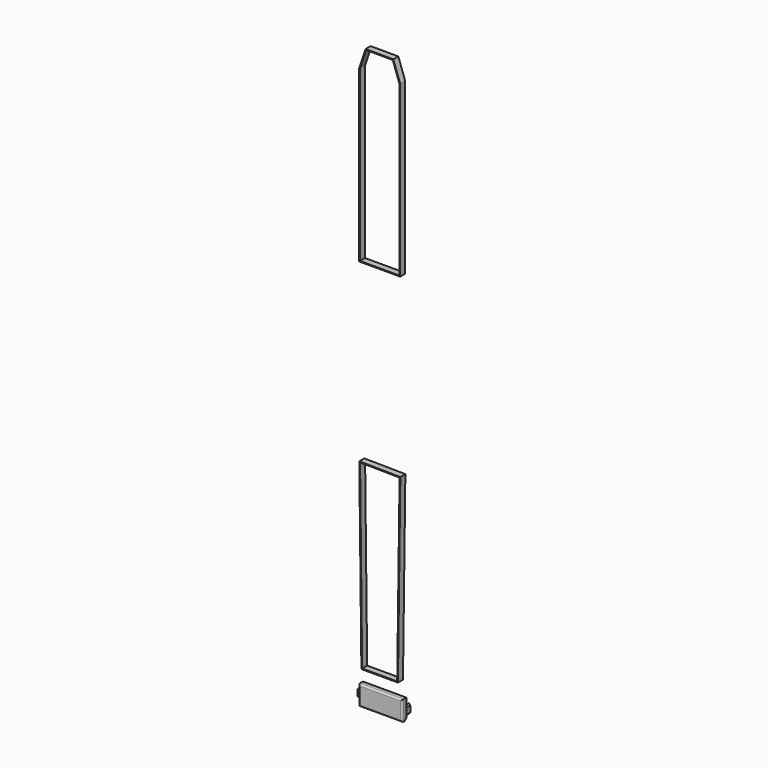
from build123d import *

# Parameters (mm, degrees)
F3_DEPTH       = 10.16
F5_DEPTH       = 10.16
F6_DEPTH       = 3.048
F7_W           = 70.5953985453
F7_H           = 32.1978032589
F8_DEPTH       = 10.16
F9_SIZE        = 5.08
F10_SIZE       = 1.778
F11_R          = 2.54
F12_T1_DEPTH   = 41.1774884869
F12_2_T1_DEPTH = 41.1774884869


# Not quite as in the source:
# - a fillet or chamfer that OpenCascade refuses, or shapes differently, is made with other operations: its cross-section is extruded or revolved along the edge and cut away or added


with BuildPart() as f3:
    # F2 (on offset) → F3 (new body)
    with BuildSketch(Plane.XZ.offset(-43.18)):
        Polygon((-35.3846980661, 135.4740036093), (30.9212480387, 135.4740036093), (30.9212480387, 410.4879885195), (19.851437657, 441.7302218888), (-0.0477681745, 441.8133852342), (-25.0969552653, 441.9180715325), (-35.3846980661, 411.4112124139), align=None)
        Polygon((29.6512480387, 410.2696444457), (29.6512480387, 136.7440036093), (-34.1146980661, 136.7440036093), (-34.1146980661, 411.2028378599), (-24.1862514864, 440.6442544017), (-0.0530757494, 440.5433963249), (18.9527356185, 440.46396668), align=None, mode=Mode.SUBTRACT)
    extrude(amount=F3_DEPTH)

    # F2 (on offset) → F6 (join)
    with BuildSketch(Plane.XZ.offset(-43.18)):
        Polygon((-35.3846980661, 135.4740036093), (30.9212480387, 135.4740036093), (30.9212480387, 410.4879885195), (19.851437657, 441.7302218888), (-0.0477681745, 441.8133852342), (-25.0969552653, 441.9180715325), (-35.3846980661, 411.4112124139), align=None)
        Polygon((29.6512480387, 410.2696444457), (29.6512480387, 136.7440036093), (-34.1146980661, 136.7440036093), (-34.1146980661, 411.2028378599), (-24.1862514864, 440.6442544017), (-0.0530757494, 440.5433963249), (18.9527356185, 440.46396668), align=None, mode=Mode.SUBTRACT)
    extrude(amount=F6_DEPTH)


with BuildPart() as f5:
    # F4 (on offset) → F5 (new body)
    with BuildSketch(Plane.XZ.offset(-43.18)):
        Polygon((27.3243936069, -444.5440577507), (31.1871017119, -150.1536065675), (-35.3159089358, -149.281018081), (-31.9307609946, -444.5440577507), (0.0040204088, -444.5440577507), align=None)
        Polygon((0.0040204088, -443.2740577507), (-30.6752378969, -443.2740577507), (-34.0310705739, -150.567985811), (29.9005487372, -151.4068349758), (26.0709480064, -443.2740577507), align=None, mode=Mode.SUBTRACT)
    extrude(amount=F5_DEPTH)


with BuildPart() as f8:
    # F7 (on offset) → F8 (new body)
    with BuildSketch(Plane.XZ.offset(-43.18)):
        with Locations((-1.0061189532, -483.1268042326)):
            Rectangle(F7_W, F7_H)
    extrude(amount=F8_DEPTH)

    # F9
    f9_edges = [f8.edges().sort_by_distance(p)[0] for p in [
        (-1.006119, 43.18, -499.225706),
    ]]
    chamfer(f9_edges, length=F9_SIZE)

    # F10
    f10_edges = [f8.edges().sort_by_distance(p)[0] for p in [
        (34.29158, 43.18, -480.586804),
        (-1.006119, 43.18, -467.027903),
        (-36.303818, 43.18, -480.586804),
    ]]
    chamfer(f10_edges, length=F10_SIZE)

    # F11
    f11_edges = [f8.edges().sort_by_distance(p)[0] for p in [
        (-1.006119, 33.02, -467.027903),
        (-36.303818, 33.02, -483.126804),
        (-1.006119, 33.02, -499.225706),
        (34.29158, 33.02, -483.126804),
    ]]
    fillet(f11_edges, radius=F11_R)


with BuildPart() as f8b:
    # F7 (on offset) → F8, piece 2 (new body)
    with BuildSketch(Plane.XZ.offset(-43.18)):
        Polygon((-38.5682731867, -489.7837042809), (-38.5682731867, -474.7345149517), (-40.443841368, -477.3021042347), (-40.443841368, -487.5218868256), align=None)
    extrude(amount=F8_DEPTH)

    # F12#2: chamfer of 5.08 on 1 edges, made by hand

    # F12_2_s2 → F12_2_t1 (cut)
    with BuildSketch(Plane.XY.offset(-502.8478538597)):
        Polygon((-38.5682731867, 38.1), (-43.6482731867, 33.02), (-38.5682731867, 33.02), align=None)
    extrude(amount=F12_2_T1_DEPTH, mode=Mode.SUBTRACT)


with BuildPart() as f8c:
    # F7 (on offset) → F8, piece 3 (new body)
    with BuildSketch(Plane.XZ.offset(-43.18)):
        Polygon((36.9912497699, -474.7345149517), (36.9912497699, -489.7837042809), (39.1628630459, -487.5218868256), (39.1628630459, -477.3021042347), align=None)
    extrude(amount=F8_DEPTH)

    # F12: chamfer of 5.08 on 1 edges, made by hand

    # F12_s2 → F12_t1 (cut)
    with BuildSketch(Plane.XY.offset(-502.8478538597)):
        Polygon((36.9912497699, 38.1), (42.0712497699, 33.02), (36.9912497699, 33.02), align=None)
    extrude(amount=F12_T1_DEPTH, mode=Mode.SUBTRACT)


solid = Compound([f3.part, f5.part, f8.part, f8b.part, f8c.part])
